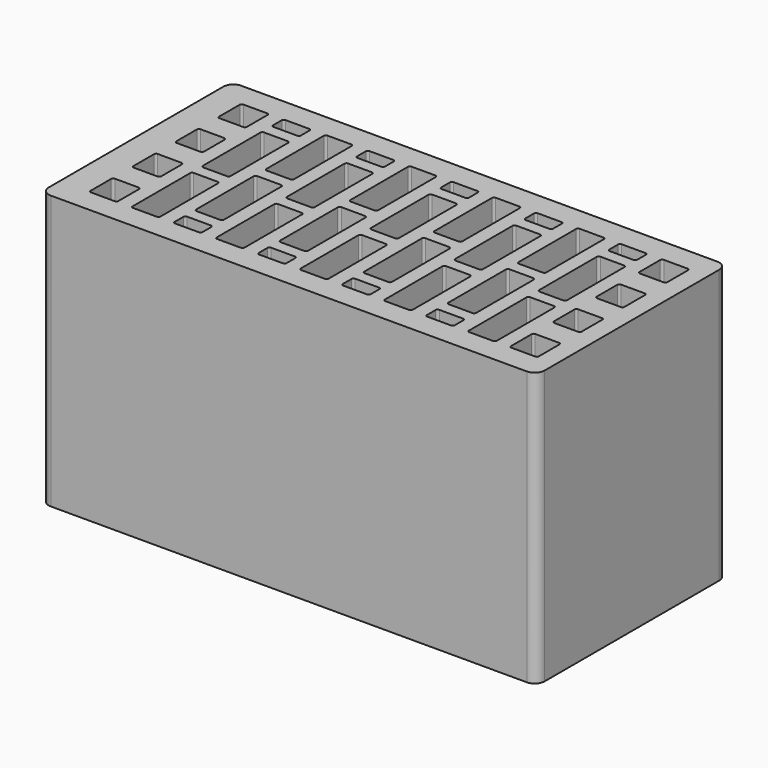
from build123d import *

# Parameters (mm, degrees)
F1_DEPTH = 138
F3_DEPTH = 138.001


# Not quite as in the source:
# - a feature names something its author has since deleted; it is built from what else it names


with BuildPart() as f1:
    # F0 (on Top) → F1 (new body)
    with BuildSketch(Plane.XY):
        with BuildLine():
            ThreePointArc((125, 55), (123.5355339059, 58.5355339059), (120, 60))
            Line((120, 60), (-120, 60))
            ThreePointArc((-120, 60), (-123.5355339059, 58.5355339059), (-125, 55))
            Line((-125, 55), (-125, -55))
            ThreePointArc((-125, -55), (-123.5355339059, -58.5355339059), (-120, -60))
            Line((-120, -60), (120, -60))
            ThreePointArc((120, -60), (123.5355339059, -58.5355339059), (125, -55))
            Line((125, -55), (125, 55))
        make_face()
        with BuildLine():
            Line((-109.336699307, -33), (-97.336699307, -33))
            ThreePointArc((-97.336699307, -33), (-96.6295925258, -33.2928932188), (-96.336699307, -34))
            Line((-96.336699307, -34), (-96.336699307, -47))
            ThreePointArc((-96.336699307, -47), (-96.6295925258, -47.7071067812), (-97.336699307, -48))
            Line((-97.336699307, -48), (-109.336699307, -48))
            ThreePointArc((-109.336699307, -48), (-110.0438060882, -47.7071067812), (-110.336699307, -47))
            Line((-110.336699307, -47), (-110.336699307, -34))
            ThreePointArc((-110.336699307, -34), (-110.0438060882, -33.2928932188), (-109.336699307, -33))
        make_face(mode=Mode.SUBTRACT)
        with BuildLine():
            Line((-109.336699307, -6), (-97.336699307, -6))
            ThreePointArc((-97.336699307, -6), (-96.6295925258, -6.2928932188), (-96.336699307, -7))
            Line((-96.336699307, -7), (-96.336699307, -20))
            ThreePointArc((-96.336699307, -20), (-96.6295925258, -20.7071067812), (-97.336699307, -21))
            Line((-97.336699307, -21), (-109.336699307, -21))
            ThreePointArc((-109.336699307, -21), (-110.0438060882, -20.7071067812), (-110.336699307, -20))
            Line((-110.336699307, -20), (-110.336699307, -7))
            ThreePointArc((-110.336699307, -7), (-110.0438060882, -6.2928932188), (-109.336699307, -6))
        make_face(mode=Mode.SUBTRACT)
        with BuildLine():
            Line((102.663300693, -33), (114.663300693, -33))
            ThreePointArc((114.663300693, -33), (115.3704074742, -33.2928932188), (115.663300693, -34))
            Line((115.663300693, -34), (115.663300693, -47))
            ThreePointArc((115.663300693, -47), (115.3704074742, -47.7071067812), (114.663300693, -48))
            Line((114.663300693, -48), (102.663300693, -48))
            ThreePointArc((102.663300693, -48), (101.9561939118, -47.7071067812), (101.663300693, -47))
            Line((101.663300693, -47), (101.663300693, -34))
            ThreePointArc((101.663300693, -34), (101.9561939118, -33.2928932188), (102.663300693, -33))
        make_face(mode=Mode.SUBTRACT)
        with BuildLine():
            Line((102.663300693, -6), (114.663300693, -6))
            ThreePointArc((114.663300693, -6), (115.3704074742, -6.2928932188), (115.663300693, -7))
            Line((115.663300693, -7), (115.663300693, -20))
            ThreePointArc((115.663300693, -20), (115.3704074742, -20.7071067812), (114.663300693, -21))
            Line((114.663300693, -21), (102.663300693, -21))
            ThreePointArc((102.663300693, -21), (101.9561939118, -20.7071067812), (101.663300693, -20))
            Line((101.663300693, -20), (101.663300693, -7))
            ThreePointArc((101.663300693, -7), (101.9561939118, -6.2928932188), (102.663300693, -6))
        make_face(mode=Mode.SUBTRACT)
        with BuildLine():
            Line((-109.336699307, 21), (-97.336699307, 21))
            ThreePointArc((-97.336699307, 21), (-96.6295925258, 20.7071067812), (-96.336699307, 20))
            Line((-96.336699307, 20), (-96.336699307, 7))
            ThreePointArc((-96.336699307, 7), (-96.6295925258, 6.2928932188), (-97.336699307, 6))
            Line((-97.336699307, 6), (-109.336699307, 6))
            ThreePointArc((-109.336699307, 6), (-110.0438060882, 6.2928932188), (-110.336699307, 7))
            Line((-110.336699307, 7), (-110.336699307, 20))
            ThreePointArc((-110.336699307, 20), (-110.0438060882, 20.7071067812), (-109.336699307, 21))
        make_face(mode=Mode.SUBTRACT)
        with BuildLine():
            Line((-109.336699307, 48), (-97.336699307, 48))
            ThreePointArc((-97.336699307, 48), (-96.6295925258, 47.7071067812), (-96.336699307, 47))
            Line((-96.336699307, 47), (-96.336699307, 34))
            ThreePointArc((-96.336699307, 34), (-96.6295925258, 33.2928932188), (-97.336699307, 33))
            Line((-97.336699307, 33), (-109.336699307, 33))
            ThreePointArc((-109.336699307, 33), (-110.0438060882, 33.2928932188), (-110.336699307, 34))
            Line((-110.336699307, 34), (-110.336699307, 47))
            ThreePointArc((-110.336699307, 47), (-110.0438060882, 47.7071067812), (-109.336699307, 48))
        make_face(mode=Mode.SUBTRACT)
        with BuildLine():
            Line((102.663300693, 21), (114.663300693, 21))
            ThreePointArc((114.663300693, 21), (115.3704074742, 20.7071067812), (115.663300693, 20))
            Line((115.663300693, 20), (115.663300693, 7))
            ThreePointArc((115.663300693, 7), (115.3704074742, 6.2928932188), (114.663300693, 6))
            Line((114.663300693, 6), (102.663300693, 6))
            ThreePointArc((102.663300693, 6), (101.9561939118, 6.2928932188), (101.663300693, 7))
            Line((101.663300693, 7), (101.663300693, 20))
            ThreePointArc((101.663300693, 20), (101.9561939118, 20.7071067812), (102.663300693, 21))
        make_face(mode=Mode.SUBTRACT)
        with BuildLine():
            Line((102.663300693, 48), (114.663300693, 48))
            ThreePointArc((114.663300693, 48), (115.3704074742, 47.7071067812), (115.663300693, 47))
            Line((115.663300693, 47), (115.663300693, 34))
            ThreePointArc((115.663300693, 34), (115.3704074742, 33.2928932188), (114.663300693, 33))
            Line((114.663300693, 33), (102.663300693, 33))
            ThreePointArc((102.663300693, 33), (101.9561939118, 33.2928932188), (101.663300693, 34))
            Line((101.663300693, 34), (101.663300693, 47))
            ThreePointArc((101.663300693, 47), (101.9561939118, 47.7071067812), (102.663300693, 48))
        make_face(mode=Mode.SUBTRACT)
    extrude(amount=F1_DEPTH)

    # F2 (on face) → F3 (cut, through all)
    with BuildSketch(Plane.XY.offset(138)):
        with BuildLine():
            ThreePointArc((-75.136699307, -10.75), (-75.4295925258, -10.0428932188), (-76.136699307, -9.75))
            Line((-76.136699307, -9.75), (-88.136699307, -9.75))
            ThreePointArc((-88.136699307, -9.75), (-88.8438060882, -10.0428932188), (-89.136699307, -10.75))
            Line((-89.136699307, -10.75), (-89.136699307, -47))
            ThreePointArc((-89.136699307, -47), (-88.8438060882, -47.7071067812), (-88.136699307, -48))
            Line((-88.136699307, -48), (-76.136699307, -48))
            ThreePointArc((-76.136699307, -48), (-75.4295925258, -47.7071067812), (-75.136699307, -47))
            Line((-75.136699307, -47), (-75.136699307, -10.75))
        make_face()
        with BuildLine():
            ThreePointArc((-75.136699307, 33.5), (-75.4295925258, 34.2071067812), (-76.136699307, 34.5))
            Line((-76.136699307, 34.5), (-88.136699307, 34.5))
            ThreePointArc((-88.136699307, 34.5), (-88.8438060882, 34.2071067812), (-89.136699307, 33.5))
            Line((-89.136699307, 33.5), (-89.136699307, -2.75))
            ThreePointArc((-89.136699307, -2.75), (-88.8438060882, -3.4571067812), (-88.136699307, -3.75))
            Line((-88.136699307, -3.75), (-76.136699307, -3.75))
            ThreePointArc((-76.136699307, -3.75), (-75.4295925258, -3.4571067812), (-75.136699307, -2.75))
            Line((-75.136699307, -2.75), (-75.136699307, 33.5))
        make_face()
        with BuildLine():
            ThreePointArc((-75.136699307, 47), (-75.4295925258, 47.7071067812), (-76.136699307, 48))
            Line((-76.136699307, 48), (-88.136699307, 48))
            ThreePointArc((-88.136699307, 48), (-88.8438060882, 47.7071067812), (-89.136699307, 47))
            Line((-89.136699307, 47), (-89.136699307, 41.5))
            ThreePointArc((-89.136699307, 41.5), (-88.8438060882, 40.7928932188), (-88.136699307, 40.5))
            Line((-88.136699307, 40.5), (-76.136699307, 40.5))
            ThreePointArc((-76.136699307, 40.5), (-75.4295925258, 40.7928932188), (-75.136699307, 41.5))
            Line((-75.136699307, 41.5), (-75.136699307, 47))
        make_face()
        with BuildLine():
            ThreePointArc((-67.936699307, 10.75), (-67.6438060882, 10.0428932188), (-66.936699307, 9.75))
            Line((-66.936699307, 9.75), (-54.936699307, 9.75))
            ThreePointArc((-54.936699307, 9.75), (-54.2295925258, 10.0428932188), (-53.936699307, 10.75))
            Line((-53.936699307, 10.75), (-53.936699307, 47))
            ThreePointArc((-53.936699307, 47), (-54.2295925258, 47.7071067812), (-54.936699307, 48))
            Line((-54.936699307, 48), (-66.936699307, 48))
            ThreePointArc((-66.936699307, 48), (-67.6438060882, 47.7071067812), (-67.936699307, 47))
            Line((-67.936699307, 47), (-67.936699307, 10.75))
        make_face()
        with BuildLine():
            ThreePointArc((-67.936699307, -33.5), (-67.6438060882, -34.2071067812), (-66.936699307, -34.5))
            Line((-66.936699307, -34.5), (-54.936699307, -34.5))
            ThreePointArc((-54.936699307, -34.5), (-54.2295925258, -34.2071067812), (-53.936699307, -33.5))
            Line((-53.936699307, -33.5), (-53.936699307, 2.75))
            ThreePointArc((-53.936699307, 2.75), (-54.2295925258, 3.4571067812), (-54.936699307, 3.75))
            Line((-54.936699307, 3.75), (-66.936699307, 3.75))
            ThreePointArc((-66.936699307, 3.75), (-67.6438060882, 3.4571067812), (-67.936699307, 2.75))
            Line((-67.936699307, 2.75), (-67.936699307, -33.5))
        make_face()
        with BuildLine():
            ThreePointArc((-67.936699307, -47), (-67.6438060882, -47.7071067812), (-66.936699307, -48))
            Line((-66.936699307, -48), (-54.936699307, -48))
            ThreePointArc((-54.936699307, -48), (-54.2295925258, -47.7071067812), (-53.936699307, -47))
            Line((-53.936699307, -47), (-53.936699307, -41.5))
            ThreePointArc((-53.936699307, -41.5), (-54.2295925258, -40.7928932188), (-54.936699307, -40.5))
            Line((-54.936699307, -40.5), (-66.936699307, -40.5))
            ThreePointArc((-66.936699307, -40.5), (-67.6438060882, -40.7928932188), (-67.936699307, -41.5))
            Line((-67.936699307, -41.5), (-67.936699307, -47))
        make_face()
        with BuildLine():
            Line((-45.736699307, -3.75), (-33.736699307, -3.75))
            ThreePointArc((-33.736699307, -3.75), (-33.0295925258, -3.4571067812), (-32.736699307, -2.75))
            Line((-32.736699307, -2.75), (-32.736699307, 33.5))
            ThreePointArc((-32.736699307, 33.5), (-33.0295925258, 34.2071067812), (-33.736699307, 34.5))
            Line((-33.736699307, 34.5), (-45.736699307, 34.5))
            ThreePointArc((-45.736699307, 34.5), (-46.4438060882, 34.2071067812), (-46.736699307, 33.5))
            Line((-46.736699307, 33.5), (-46.736699307, -2.75))
            ThreePointArc((-46.736699307, -2.75), (-46.4438060882, -3.4571067812), (-45.736699307, -3.75))
        make_face()
        with BuildLine():
            Line((-45.736699307, 40.5), (-33.736699307, 40.5))
            ThreePointArc((-33.736699307, 40.5), (-33.0295925258, 40.7928932188), (-32.736699307, 41.5))
            Line((-32.736699307, 41.5), (-32.736699307, 47))
            ThreePointArc((-32.736699307, 47), (-33.0295925258, 47.7071067812), (-33.736699307, 48))
            Line((-33.736699307, 48), (-45.736699307, 48))
            ThreePointArc((-45.736699307, 48), (-46.4438060882, 47.7071067812), (-46.736699307, 47))
            Line((-46.736699307, 47), (-46.736699307, 41.5))
            ThreePointArc((-46.736699307, 41.5), (-46.4438060882, 40.7928932188), (-45.736699307, 40.5))
        make_face()
        with BuildLine():
            ThreePointArc((-32.736699307, -10.75), (-33.0295925258, -10.0428932188), (-33.736699307, -9.75))
            Line((-33.736699307, -9.75), (-45.736699307, -9.75))
            ThreePointArc((-45.736699307, -9.75), (-46.4438060882, -10.0428932188), (-46.736699307, -10.75))
            Line((-46.736699307, -10.75), (-46.736699307, -47))
            ThreePointArc((-46.736699307, -47), (-46.4438060882, -47.7071067812), (-45.736699307, -48))
            Line((-45.736699307, -48), (-33.736699307, -48))
            ThreePointArc((-33.736699307, -48), (-33.0295925258, -47.7071067812), (-32.736699307, -47))
            Line((-32.736699307, -47), (-32.736699307, -10.75))
        make_face()
        with BuildLine():
            ThreePointArc((-25.536699307, -47), (-25.2438060882, -47.7071067812), (-24.536699307, -48))
            Line((-24.536699307, -48), (-12.536699307, -48))
            ThreePointArc((-12.536699307, -48), (-11.8295925258, -47.7071067812), (-11.536699307, -47))
            Line((-11.536699307, -47), (-11.536699307, -41.5))
            ThreePointArc((-11.536699307, -41.5), (-11.8295925258, -40.7928932188), (-12.536699307, -40.5))
            Line((-12.536699307, -40.5), (-24.536699307, -40.5))
            ThreePointArc((-24.536699307, -40.5), (-25.2438060882, -40.7928932188), (-25.536699307, -41.5))
            Line((-25.536699307, -41.5), (-25.536699307, -47))
        make_face()
        with BuildLine():
            ThreePointArc((-25.536699307, -33.5), (-25.2438060882, -34.2071067812), (-24.536699307, -34.5))
            Line((-24.536699307, -34.5), (-12.536699307, -34.5))
            ThreePointArc((-12.536699307, -34.5), (-11.8295925258, -34.2071067812), (-11.536699307, -33.5))
            Line((-11.536699307, -33.5), (-11.536699307, 2.75))
            ThreePointArc((-11.536699307, 2.75), (-11.8295925258, 3.4571067812), (-12.536699307, 3.75))
            Line((-12.536699307, 3.75), (-24.536699307, 3.75))
            ThreePointArc((-24.536699307, 3.75), (-25.2438060882, 3.4571067812), (-25.536699307, 2.75))
            Line((-25.536699307, 2.75), (-25.536699307, -33.5))
        make_face()
        with BuildLine():
            Line((-25.536699307, 47), (-25.536699307, 10.75))
            ThreePointArc((-25.536699307, 10.75), (-25.2438060882, 10.0428932188), (-24.536699307, 9.75))
            Line((-24.536699307, 9.75), (-12.536699307, 9.75))
            ThreePointArc((-12.536699307, 9.75), (-11.8295925258, 10.0428932188), (-11.536699307, 10.75))
            Line((-11.536699307, 10.75), (-11.536699307, 47))
            ThreePointArc((-11.536699307, 47), (-11.8295925258, 47.7071067812), (-12.536699307, 48))
            Line((-12.536699307, 48), (-24.536699307, 48))
            ThreePointArc((-24.536699307, 48), (-25.2438060882, 47.7071067812), (-25.536699307, 47))
        make_face()
        with BuildLine():
            Line((-3.336699307, 40.5), (8.663300693, 40.5))
            ThreePointArc((8.663300693, 40.5), (9.3704074742, 40.7928932188), (9.663300693, 41.5))
            Line((9.663300693, 41.5), (9.663300693, 47))
            ThreePointArc((9.663300693, 47), (9.3704074742, 47.7071067812), (8.663300693, 48))
            Line((8.663300693, 48), (-3.336699307, 48))
            ThreePointArc((-3.336699307, 48), (-4.0438060882, 47.7071067812), (-4.336699307, 47))
            Line((-4.336699307, 47), (-4.336699307, 41.5))
            ThreePointArc((-4.336699307, 41.5), (-4.0438060882, 40.7928932188), (-3.336699307, 40.5))
        make_face()
        with BuildLine():
            Line((-3.336699307, -3.75), (8.663300693, -3.75))
            ThreePointArc((8.663300693, -3.75), (9.3704074742, -3.4571067812), (9.663300693, -2.75))
            Line((9.663300693, -2.75), (9.663300693, 33.5))
            ThreePointArc((9.663300693, 33.5), (9.3704074742, 34.2071067812), (8.663300693, 34.5))
            Line((8.663300693, 34.5), (-3.336699307, 34.5))
            ThreePointArc((-3.336699307, 34.5), (-4.0438060882, 34.2071067812), (-4.336699307, 33.5))
            Line((-4.336699307, 33.5), (-4.336699307, -2.75))
            ThreePointArc((-4.336699307, -2.75), (-4.0438060882, -3.4571067812), (-3.336699307, -3.75))
        make_face()
        with BuildLine():
            ThreePointArc((9.663300693, -10.75), (9.3704074742, -10.0428932188), (8.663300693, -9.75))
            Line((8.663300693, -9.75), (-3.336699307, -9.75))
            ThreePointArc((-3.336699307, -9.75), (-4.0438060882, -10.0428932188), (-4.336699307, -10.75))
            Line((-4.336699307, -10.75), (-4.336699307, -47))
            ThreePointArc((-4.336699307, -47), (-4.0438060882, -47.7071067812), (-3.336699307, -48))
            Line((-3.336699307, -48), (8.663300693, -48))
            ThreePointArc((8.663300693, -48), (9.3704074742, -47.7071067812), (9.663300693, -47))
            Line((9.663300693, -47), (9.663300693, -10.75))
        make_face()
        with BuildLine():
            ThreePointArc((16.863300693, -33.5), (17.1561939118, -34.2071067812), (17.863300693, -34.5))
            Line((17.863300693, -34.5), (29.863300693, -34.5))
            ThreePointArc((29.863300693, -34.5), (30.5704074742, -34.2071067812), (30.863300693, -33.5))
            Line((30.863300693, -33.5), (30.863300693, 2.75))
            ThreePointArc((30.863300693, 2.75), (30.5704074742, 3.4571067812), (29.863300693, 3.75))
            Line((29.863300693, 3.75), (17.863300693, 3.75))
            ThreePointArc((17.863300693, 3.75), (17.1561939118, 3.4571067812), (16.863300693, 2.75))
            Line((16.863300693, 2.75), (16.863300693, -33.5))
        make_face()
        with BuildLine():
            ThreePointArc((16.863300693, -47), (17.1561939118, -47.7071067812), (17.863300693, -48))
            Line((17.863300693, -48), (29.863300693, -48))
            ThreePointArc((29.863300693, -48), (30.5704074742, -47.7071067812), (30.863300693, -47))
            Line((30.863300693, -47), (30.863300693, -41.5))
            ThreePointArc((30.863300693, -41.5), (30.5704074742, -40.7928932188), (29.863300693, -40.5))
            Line((29.863300693, -40.5), (17.863300693, -40.5))
            ThreePointArc((17.863300693, -40.5), (17.1561939118, -40.7928932188), (16.863300693, -41.5))
            Line((16.863300693, -41.5), (16.863300693, -47))
        make_face()
        with BuildLine():
            Line((16.863300693, 47), (16.863300693, 10.75))
            ThreePointArc((16.863300693, 10.75), (17.1561939118, 10.0428932188), (17.863300693, 9.75))
            Line((17.863300693, 9.75), (29.863300693, 9.75))
            ThreePointArc((29.863300693, 9.75), (30.5704074742, 10.0428932188), (30.863300693, 10.75))
            Line((30.863300693, 10.75), (30.863300693, 47))
            ThreePointArc((30.863300693, 47), (30.5704074742, 47.7071067812), (29.863300693, 48))
            Line((29.863300693, 48), (17.863300693, 48))
            ThreePointArc((17.863300693, 48), (17.1561939118, 47.7071067812), (16.863300693, 47))
        make_face()
        with BuildLine():
            Line((39.063300693, 40.5), (51.063300693, 40.5))
            ThreePointArc((51.063300693, 40.5), (51.7704074742, 40.7928932188), (52.063300693, 41.5))
            Line((52.063300693, 41.5), (52.063300693, 47))
            ThreePointArc((52.063300693, 47), (51.7704074742, 47.7071067812), (51.063300693, 48))
            Line((51.063300693, 48), (39.063300693, 48))
            ThreePointArc((39.063300693, 48), (38.3561939118, 47.7071067812), (38.063300693, 47))
            Line((38.063300693, 47), (38.063300693, 41.5))
            ThreePointArc((38.063300693, 41.5), (38.3561939118, 40.7928932188), (39.063300693, 40.5))
        make_face()
        with BuildLine():
            Line((39.063300693, -3.75), (51.063300693, -3.75))
            ThreePointArc((51.063300693, -3.75), (51.7704074742, -3.4571067812), (52.063300693, -2.75))
            Line((52.063300693, -2.75), (52.063300693, 33.5))
            ThreePointArc((52.063300693, 33.5), (51.7704074742, 34.2071067812), (51.063300693, 34.5))
            Line((51.063300693, 34.5), (39.063300693, 34.5))
            ThreePointArc((39.063300693, 34.5), (38.3561939118, 34.2071067812), (38.063300693, 33.5))
            Line((38.063300693, 33.5), (38.063300693, -2.75))
            ThreePointArc((38.063300693, -2.75), (38.3561939118, -3.4571067812), (39.063300693, -3.75))
        make_face()
        with BuildLine():
            ThreePointArc((52.063300693, -10.75), (51.7704074742, -10.0428932188), (51.063300693, -9.75))
            Line((51.063300693, -9.75), (39.063300693, -9.75))
            ThreePointArc((39.063300693, -9.75), (38.3561939118, -10.0428932188), (38.063300693, -10.75))
            Line((38.063300693, -10.75), (38.063300693, -47))
            ThreePointArc((38.063300693, -47), (38.3561939118, -47.7071067812), (39.063300693, -48))
            Line((39.063300693, -48), (51.063300693, -48))
            ThreePointArc((51.063300693, -48), (51.7704074742, -47.7071067812), (52.063300693, -47))
            Line((52.063300693, -47), (52.063300693, -10.75))
        make_face()
        with BuildLine():
            ThreePointArc((59.263300693, -33.5), (59.5561939118, -34.2071067812), (60.263300693, -34.5))
            Line((60.263300693, -34.5), (72.263300693, -34.5))
            ThreePointArc((72.263300693, -34.5), (72.9704074742, -34.2071067812), (73.263300693, -33.5))
            Line((73.263300693, -33.5), (73.263300693, 2.75))
            ThreePointArc((73.263300693, 2.75), (72.9704074742, 3.4571067812), (72.263300693, 3.75))
            Line((72.263300693, 3.75), (60.263300693, 3.75))
            ThreePointArc((60.263300693, 3.75), (59.5561939118, 3.4571067812), (59.263300693, 2.75))
            Line((59.263300693, 2.75), (59.263300693, -33.5))
        make_face()
        with BuildLine():
            Line((59.263300693, 47), (59.263300693, 10.75))
            ThreePointArc((59.263300693, 10.75), (59.5561939118, 10.0428932188), (60.263300693, 9.75))
            Line((60.263300693, 9.75), (72.263300693, 9.75))
            ThreePointArc((72.263300693, 9.75), (72.9704074742, 10.0428932188), (73.263300693, 10.75))
            Line((73.263300693, 10.75), (73.263300693, 47))
            ThreePointArc((73.263300693, 47), (72.9704074742, 47.7071067812), (72.263300693, 48))
            Line((72.263300693, 48), (60.263300693, 48))
            ThreePointArc((60.263300693, 48), (59.5561939118, 47.7071067812), (59.263300693, 47))
        make_face()
        with BuildLine():
            Line((81.463300693, 40.5), (93.463300693, 40.5))
            ThreePointArc((93.463300693, 40.5), (94.1704074742, 40.7928932188), (94.463300693, 41.5))
            Line((94.463300693, 41.5), (94.463300693, 47))
            ThreePointArc((94.463300693, 47), (94.1704074742, 47.7071067812), (93.463300693, 48))
            Line((93.463300693, 48), (81.463300693, 48))
            ThreePointArc((81.463300693, 48), (80.7561939118, 47.7071067812), (80.463300693, 47))
            Line((80.463300693, 47), (80.463300693, 41.5))
            ThreePointArc((80.463300693, 41.5), (80.7561939118, 40.7928932188), (81.463300693, 40.5))
        make_face()
        with BuildLine():
            Line((81.463300693, -3.75), (93.463300693, -3.75))
            ThreePointArc((93.463300693, -3.75), (94.1704074742, -3.4571067812), (94.463300693, -2.75))
            Line((94.463300693, -2.75), (94.463300693, 33.5))
            ThreePointArc((94.463300693, 33.5), (94.1704074742, 34.2071067812), (93.463300693, 34.5))
            Line((93.463300693, 34.5), (81.463300693, 34.5))
            ThreePointArc((81.463300693, 34.5), (80.7561939118, 34.2071067812), (80.463300693, 33.5))
            Line((80.463300693, 33.5), (80.463300693, -2.75))
            ThreePointArc((80.463300693, -2.75), (80.7561939118, -3.4571067812), (81.463300693, -3.75))
        make_face()
        with BuildLine():
            ThreePointArc((94.463300693, -10.75), (94.1704074742, -10.0428932188), (93.463300693, -9.75))
            Line((93.463300693, -9.75), (81.463300693, -9.75))
            ThreePointArc((81.463300693, -9.75), (80.7561939118, -10.0428932188), (80.463300693, -10.75))
            Line((80.463300693, -10.75), (80.463300693, -47))
            ThreePointArc((80.463300693, -47), (80.7561939118, -47.7071067812), (81.463300693, -48))
            Line((81.463300693, -48), (93.463300693, -48))
            ThreePointArc((93.463300693, -48), (94.1704074742, -47.7071067812), (94.463300693, -47))
            Line((94.463300693, -47), (94.463300693, -10.75))
        make_face()
        with BuildLine():
            ThreePointArc((59.263300693, -47), (59.5561939118, -47.7071067812), (60.263300693, -48))
            Line((60.263300693, -48), (72.263300693, -48))
            ThreePointArc((72.263300693, -48), (72.9704074742, -47.7071067812), (73.263300693, -47))
            Line((73.263300693, -47), (73.263300693, -41.5))
            ThreePointArc((73.263300693, -41.5), (72.9704074742, -40.7928932188), (72.263300693, -40.5))
            Line((72.263300693, -40.5), (60.263300693, -40.5))
            ThreePointArc((60.263300693, -40.5), (59.5561939118, -40.7928932188), (59.263300693, -41.5))
            Line((59.263300693, -41.5), (59.263300693, -47))
        make_face()
    extrude(amount=-F3_DEPTH, mode=Mode.SUBTRACT)


solid = f1.part
